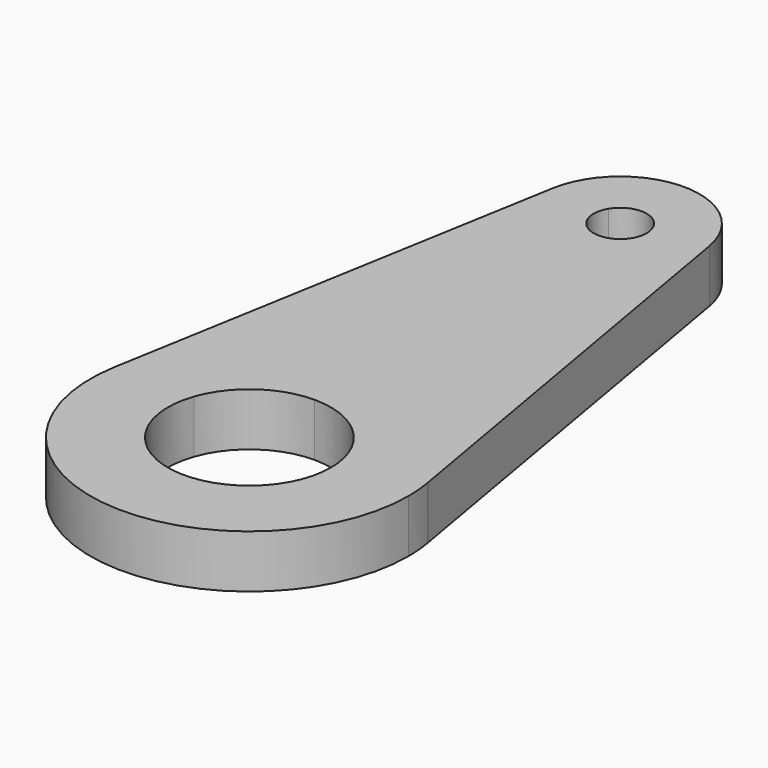
from build123d import *

# Parameters (mm, degrees)
F1_DEPTH = 6.35


with BuildPart() as f1:
    # F0 (on Top) → F1 (new body)
    with BuildSketch(Plane.XY):
        with BuildLine():
            ThreePointArc((-18.7706, 3.2507038684), (-1.6313445375, -18.98002147), (19.05, 0))
            ThreePointArc((19.05, 0), (18.98002147, 1.6313445375), (18.7706, 3.2507038684))
            Line((18.7706, 3.2507038684), (9.222893546, 3.2507038684))
            ThreePointArc((9.222893546, 3.2507038684), (9.6389708213, 1.6489640709), (9.779, 0))
            ThreePointArc((9.779, 0), (-1.6489640709, -9.6389708213), (-9.222893546, 3.2507038684))
            Line((-9.222893546, 3.2507038684), (-18.7706, 3.2507038684))
        make_face()
        with BuildLine():
            Line((-9.3853, 57.1878519342), (-18.7706, 3.2507038684))
            ThreePointArc((-18.7706, 3.2507038684), (-12.2673671036, 14.5744366734), (0, 19.05))
            Line((0, 19.05), (0, 46.0375))
            ThreePointArc((0, 46.0375), (-7.2872183367, 49.4288164482), (-9.3853, 57.1878519342))
        make_face()
        with BuildLine():
            Line((9.222893546, 3.2507038684), (18.7706, 3.2507038684))
            ThreePointArc((18.7706, 3.2507038684), (12.2673671036, 14.5744366734), (0, 19.05))
            Line((0, 19.05), (0, 9.779))
            ThreePointArc((0, 9.779), (5.6497879549, 7.9817753078), (9.222893546, 3.2507038684))
        make_face()
        with BuildLine():
            ThreePointArc((0, 19.05), (12.2673671036, 14.5744366734), (18.7706, 3.2507038684))
            Line((18.7706, 3.2507038684), (9.3853, 57.1878519342))
            ThreePointArc((9.3853, 57.1878519342), (9.490010735, 56.3781722687), (9.525, 55.5625))
            ThreePointArc((9.525, 55.5625), (6.7351920908, 48.8273079092), (0, 46.0375))
            Line((0, 46.0375), (0, 19.05))
        make_face()
        with BuildLine():
            ThreePointArc((0, 19.05), (-12.2673671036, 14.5744366734), (-18.7706, 3.2507038684))
            Line((-18.7706, 3.2507038684), (-9.222893546, 3.2507038684))
            ThreePointArc((-9.222893546, 3.2507038684), (-5.6497879549, 7.9817753078), (0, 9.779))
            Line((0, 9.779), (0, 19.05))
        make_face()
        with BuildLine():
            Line((2.7274266425, 57.1878519342), (9.3853, 57.1878519342))
            ThreePointArc((9.3853, 57.1878519342), (0, 65.0875), (-9.3853, 57.1878519342))
            Line((-9.3853, 57.1878519342), (-2.7274266425, 57.1878519342))
            ThreePointArc((-2.7274266425, 57.1878519342), (0, 58.7375), (2.7274266425, 57.1878519342))
        make_face()
        with BuildLine():
            ThreePointArc((9.525, 55.5625), (9.490010735, 56.3781722687), (9.3853, 57.1878519342))
            Line((9.3853, 57.1878519342), (2.7274266425, 57.1878519342))
            ThreePointArc((2.7274266425, 57.1878519342), (3.0610622821, 56.4054250887), (3.175, 55.5625))
            ThreePointArc((3.175, 55.5625), (2.2450640303, 53.3174359697), (0, 52.3875))
            Line((0, 52.3875), (0, 46.0375))
            ThreePointArc((0, 46.0375), (6.7351920908, 48.8273079092), (9.525, 55.5625))
        make_face()
        with BuildLine():
            Line((-2.7274266425, 57.1878519342), (-9.3853, 57.1878519342))
            ThreePointArc((-9.3853, 57.1878519342), (-7.2872183367, 49.4288164482), (0, 46.0375))
            Line((0, 46.0375), (0, 52.3875))
            ThreePointArc((0, 52.3875), (-2.7605359435, 53.9940401489), (-2.7274266425, 57.1878519342))
        make_face()
    extrude(amount=F1_DEPTH)


solid = f1.part
